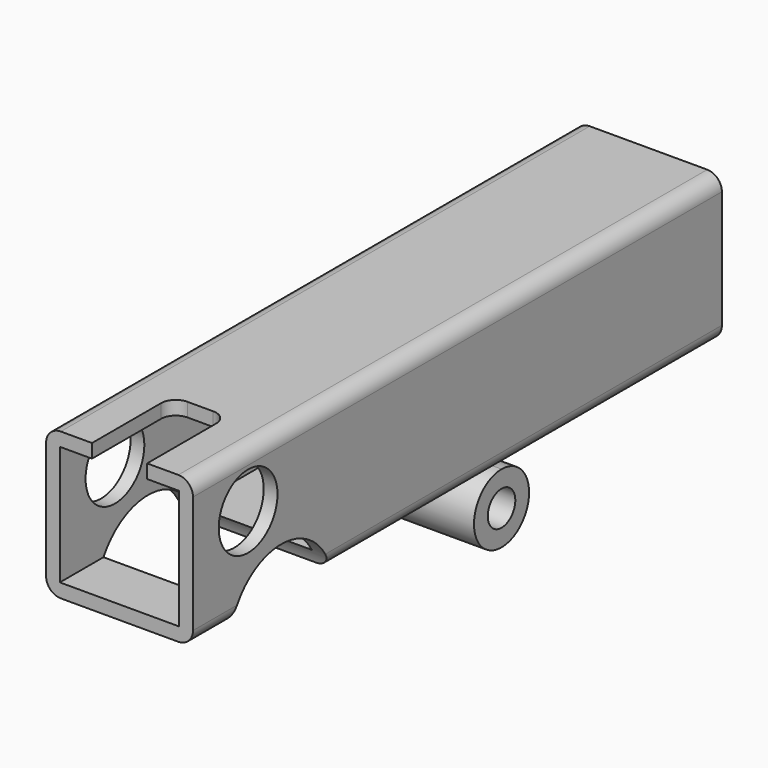
from build123d import *

# Parameters (mm, degrees)
F0_W        = 50.8
F0_H        = 50.8
F0_W_2      = 41.275
F0_H_2      = 41.275
F1_DEPTH    = 228.6
F2_R        = 22.225
F2_R_2      = 12.7
F3_DEPTH    = 25.4
F4_R        = 5.953125
F5_DEPTH    = 50.8
F6_T1_DEPTH = 254
F6_T3_DEPTH = 86.6514525143
F6_T5_DEPTH = 107.95
F6_T7_DEPTH = 42.2014525143
F7_W        = 19.05
F7_H        = 34.925
F8_DEPTH    = 4.7625
F9_R        = 5.08
F11_D       = 9.525
F11_DEPTH   = 12.7
F11_TIP     = 2.8615986981


# Not quite as in the source:
# - a fillet or chamfer that OpenCascade refuses, or shapes differently, is made with other operations: its cross-section is extruded or revolved along the edge and cut away or added


with BuildPart() as f1:
    # F0 (on Front) → F1 (new body)
    with BuildSketch(Plane.XZ):
        Rectangle(F0_W, F0_H)
        Rectangle(F0_W_2, F0_H_2, mode=Mode.SUBTRACT)
    extrude(amount=-F1_DEPTH)

    # F2 (on Right) → F3 (cut, symmetric)
    with BuildSketch(Plane.YZ):
        with Locations((38.1, -31.75)):
            Circle(F2_R)
        with Locations((23.8125, 6.35)):
            Circle(F2_R_2)
    extrude(amount=F3_DEPTH, both=True, mode=Mode.SUBTRACT)

    # F4 (on face) → F5 (join)
    with BuildSketch(Plane.YZ.offset(25.4)):
        with BuildLine():
            ThreePointArc((133.35, -25.4), (124.9310098865, -45.7252401135), (145.25625, -37.30625))
            ThreePointArc((145.25625, -37.30625), (141.7689901135, -28.8872598865), (133.35, -25.4))
        make_face()
        with Locations((133.35, -37.30625)):
            Circle(F4_R, mode=Mode.SUBTRACT)
    extrude(amount=-F5_DEPTH)

    # F6: fillet of radius 5.08 on 8 edges, made by hand

    # F6_s2 → F6_t1 (cut)
    with BuildSketch(Plane.XZ.offset(-241.3)):
        with BuildLine():
            ThreePointArc((25.4, 20.32), (23.9121024484, 23.9121024484), (20.32, 25.4))
            Line((20.32, 25.4), (25.4, 25.4))
            Line((25.4, 25.4), (25.4, 20.32))
        make_face()
        with BuildLine():
            ThreePointArc((-20.32, 25.4), (-23.9121024484, 23.9121024484), (-25.4, 20.32))
            Line((-25.4, 20.32), (-25.4, 25.4))
            Line((-25.4, 25.4), (-20.32, 25.4))
        make_face()
    extrude(amount=F6_T1_DEPTH, mode=Mode.SUBTRACT)

    # F6_s4 → F6_t3 (cut)
    with BuildSketch(Plane.XZ.offset(-133.35)):
        with BuildLine():
            ThreePointArc((25.4, -20.32), (23.9121024484, -23.9121024484), (20.32, -25.4))
            Line((20.32, -25.4), (25.4, -25.4))
            Line((25.4, -25.4), (25.4, -20.32))
        make_face()
        with BuildLine():
            ThreePointArc((-20.32, -25.4), (-23.9121024484, -23.9121024484), (-25.4, -20.32))
            Line((-25.4, -20.32), (-25.4, -25.4))
            Line((-25.4, -25.4), (-20.32, -25.4))
        make_face()
    extrude(amount=F6_T3_DEPTH, mode=Mode.SUBTRACT)

    # F6_s6 → F6_t5 (cut)
    with BuildSketch(Plane.XZ.offset(-241.3)):
        with BuildLine():
            ThreePointArc((25.4, -20.32), (23.9121024484, -23.9121024484), (20.32, -25.4))
            Line((20.32, -25.4), (25.4, -25.4))
            Line((25.4, -25.4), (25.4, -20.32))
        make_face()
        with BuildLine():
            ThreePointArc((-20.32, -25.4), (-23.9121024484, -23.9121024484), (-25.4, -20.32))
            Line((-25.4, -20.32), (-25.4, -25.4))
            Line((-25.4, -25.4), (-20.32, -25.4))
        make_face()
    extrude(amount=F6_T5_DEPTH, mode=Mode.SUBTRACT)

    # F6_s8 → F6_t7 (cut)
    with BuildSketch(Plane.XZ.offset(-29.5014525143)):
        with BuildLine():
            ThreePointArc((25.4, -20.32), (23.9121024484, -23.9121024484), (20.32, -25.4))
            Line((20.32, -25.4), (25.4, -25.4))
            Line((25.4, -25.4), (25.4, -20.32))
        make_face()
        with BuildLine():
            ThreePointArc((-20.32, -25.4), (-23.9121024484, -23.9121024484), (-25.4, -20.32))
            Line((-25.4, -20.32), (-25.4, -25.4))
            Line((-25.4, -25.4), (-20.32, -25.4))
        make_face()
    extrude(amount=F6_T7_DEPTH, mode=Mode.SUBTRACT)

    # F7 (on face) → F8 (cut, through all)
    with BuildSketch(Plane.XY.offset(25.4)):
        with Locations((0, 17.4625)):
            Rectangle(F7_W, F7_H)
    extrude(amount=-F8_DEPTH, mode=Mode.SUBTRACT)

    # F9
    f9_edges = [f1.edges().sort_by_distance(p)[0] for p in [
        (9.525, 34.925, 23.01875),
        (-9.525, 34.925, 23.01875),
    ]]
    fillet(f9_edges, radius=F9_R)

    # F11
    with Locations(Plane(origin=(-25.4, 0, 0), x_dir=(0, -1, 0), z_dir=(-1, 0, 0))):
        with Locations((-209.55, 0)):
            Hole(F11_D / 2, depth=F11_DEPTH)
            with Locations((0, 0, -(F11_DEPTH + F11_TIP / 2))):  # 118° drill point
                Cone(0, F11_D / 2, F11_TIP, mode=Mode.SUBTRACT)


solid = f1.part
